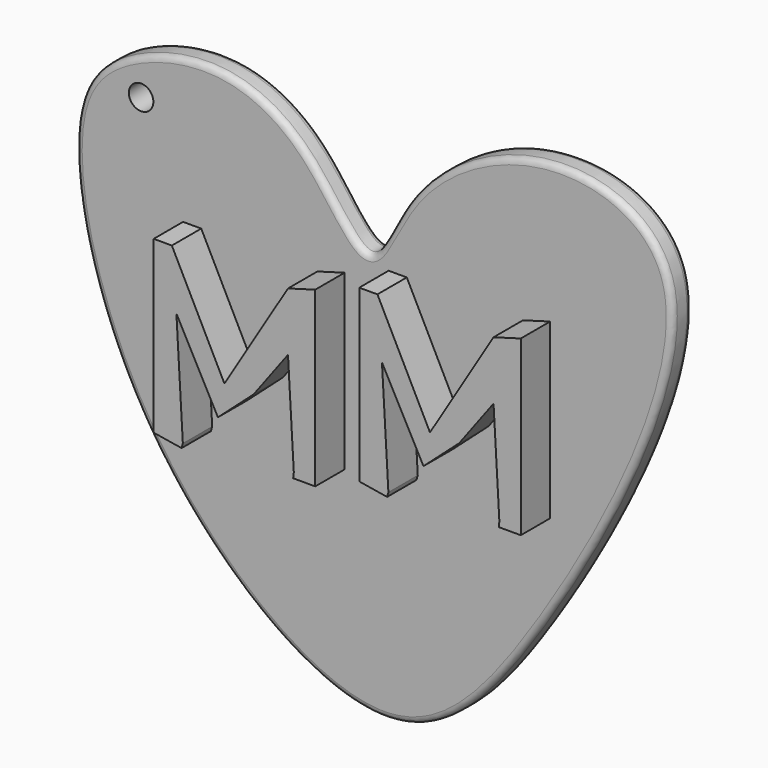
from build123d import *

# Parameters (mm, degrees)
F1_DEPTH = 3
F3_DEPTH = 2
F5_D     = 2
F6_R     = 0.5
F7_R     = 0.5


with BuildPart() as f1:
    # F0 (on Front) → F1 (new body)
    with BuildSketch(Plane.XZ):
        Polygon((-14.5881369958, 25.5385414394), (-16.0726186447, 25.5385414394), (-16.0726186447, 11.5950182185), (-13.7928792491, 11.2238978063), (-13.6912336907, 11.5950182185), (-14.2170157449, 20.7669932821), (-10.8239159513, 14.4049295617), (-7.9079695756, 17.0027722376), (-5.0980584421, 20.7669932821), (-4.6209036264, 12.4432933067), (-4.6739208281, 12.0191556927), (-2.8713361085, 12.0191556927), (-2.8713361085, 26.1747467421), (-5.0980584421, 25.5385414394), (-10.2937433747, 17.0027722376), align=None)
    extrude(amount=F1_DEPTH)



with BuildPart() as f1b:
    # F0 (on Front) → F1, piece 2 (new body)
    with BuildSketch(Plane.XZ):
        Polygon((2.2105804681, 27.4887946945), (0.7260988191, 27.4887946945), (0.7260988191, 13.5452714737), (3.0058382147, 13.1741510614), (3.1074837731, 13.5452714737), (2.581701719, 22.7172465373), (5.9748015126, 16.3551828168), (8.8907478882, 18.9530254928), (11.7006590217, 22.7172465373), (12.1778138374, 14.3935465618), (12.1247966357, 13.9694089479), (13.9273813553, 13.9694089479), (13.9273813553, 28.1249999973), (11.7006590217, 27.4887946945), (6.5049740892, 18.9530254928), align=None)
    extrude(amount=F1_DEPTH)


with BuildPart() as f1_1:
    add(f1.part)

    add(f1b.part)  # F3 merges F1b
    # F2 (on Front) → F3 (join)
    with BuildSketch(Plane.XZ):
        with BuildLine():
            add(Edge.make_bspline(
                [(0, -4.8217806034), (-5.917012886, -4.5764674848), (-21.2699337911, 7.640565446), (-26.5533504707, 30.0854088537), (-21.5746934463, 36.1504975828), (-13.1269569928, 38.4221062428), (-5.5563432865, 34.6134672931), (-0.6249960389, 25.1999046788), (2.101165727, 34.9353180936), (13.639969648, 41.5759480786), (29.5955256894, 35.2010556075), (13.5378467017, 4.3594535567), (4.9414584071, -5.0266482614), (0, -4.8217806034)],
                knots=[0, 0, 0, 0, 0.1224950399, 0.2409083717, 0.3050895141, 0.3761244596, 0.4505876323, 0.5183400151, 0.5821346978, 0.673335888, 0.757315698, 0.8977010603, 1, 1, 1, 1], degree=3))
        make_face()
    extrude(amount=-F3_DEPTH)

    # F5 (through all)
    with Locations(Plane.XZ):
        with Locations((-19.5001922548, 33.3819761872)):
            Hole(F5_D / 2)

    # F6
    f6_edges = [f1_1.edges().sort_by_distance(p)[0] for p in [
        (0.196329, 0, 29.059986),
    ]]
    fillet(f6_edges, radius=F6_R)

    # F7
    f7_edges = [f1_1.edges().sort_by_distance(p)[0] for p in [
        (0.196329, 2, 29.059986),
    ]]
    fillet(f7_edges, radius=F7_R)


solid = f1_1.part
